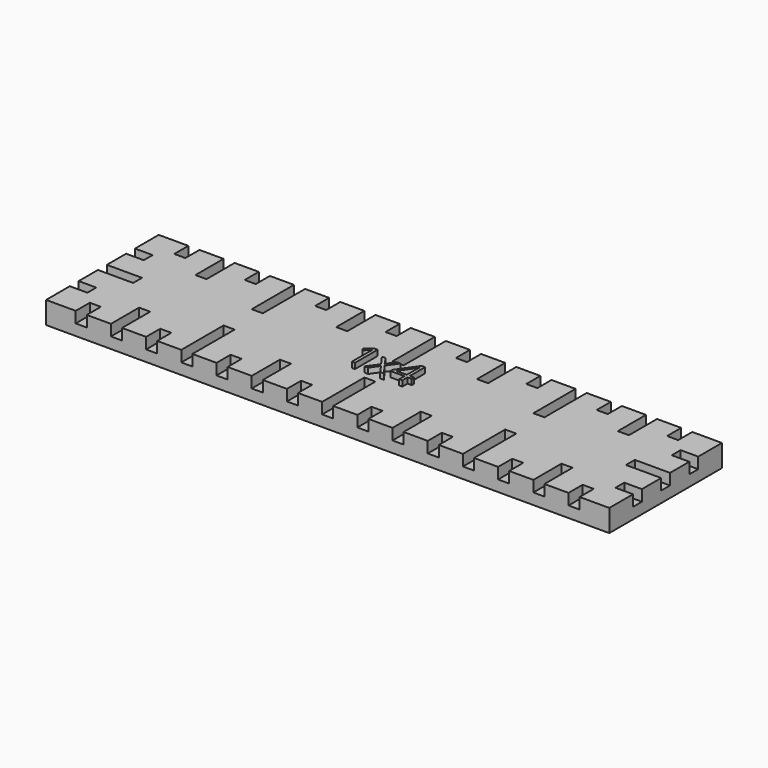
from build123d import *

# Parameters (mm, degrees)
F0_W         = 101.6
F0_H         = 25.4
F1_DEPTH     = 4
F2_W         = 2
F2_H         = 19.05
F2_H_2       = 6.35
F2_W_2       = 12.7
F2_H_3       = 2
F2_W_3       = 6.35
F2_H_4       = 12.7
F2_W_4       = 0.0030803442
F2_W_5       = 1.9969196558
F2_H_5       = 6.3500001535
F3_DEPTH     = 2
F4_TEXT_SIZE = 7.1658423015
F5_DEPTH     = 1


# Not quite as in the source:
# - ends of sketch curves that miss each other by under 0.0002 mm in the source are joined
# - Text() gives the source's letters only with a copy of the font that has no kerning and outlines rounded to 1/6400 em; it was checked with that copy


with BuildPart() as f1:
    # F0 (on Top) → F1 (new body)
    with BuildSketch(Plane.XY):
        Rectangle(F0_W, F0_H)
    extrude(amount=F1_DEPTH)

    # F2 (on face) → F3 (cut)
    with BuildSketch(Plane.XY.offset(4)):
        with Locations((0, -12.7)):
            Rectangle(F2_W, F2_H)
        with Locations((6.35, -12.7)):
            Rectangle(F2_W, F2_H_2)
        with Locations((-6.35, -12.7)):
            Rectangle(F2_W, F2_H_2)
        with Locations((-50.8, 0)):
            Rectangle(F2_W_2, F2_H_3)
        with Locations((-50.8, 6.35)):
            Rectangle(F2_W_3, F2_H_3)
        with Locations((-50.8, -6.35)):
            Rectangle(F2_W_3, F2_H_3)
        with Locations((0, 12.7)):
            Rectangle(F2_W, F2_H)
        with Locations((-6.35, 12.7)):
            Rectangle(F2_W, F2_H_2)
        with Locations((6.35, 12.7)):
            Rectangle(F2_W, F2_H_2)
        with Locations((50.8, 0)):
            Rectangle(F2_W_2, F2_H_3)
        with Locations((50.8, -6.35)):
            Rectangle(F2_W_3, F2_H_3)
        with Locations((50.8, 6.35)):
            Rectangle(F2_W_3, F2_H_3)
        with Locations((-12.7, 12.7000001177)):
            Rectangle(F2_W, F2_H_4)
        with Locations((-18.0515401721, 12.7000001177)):
            Rectangle(F2_W_4, F2_H_2)
        with Locations((-19.0515401721, 12.7000001177)):
            Rectangle(F2_W_5, F2_H_2)
        with Locations((-20.0515401721, 12.700000041)):
            Rectangle(F2_W_4, F2_H_5)
        with Locations((-12.7, -12.7000005066)):
            Rectangle(F2_W, F2_H_4)
        with Locations((-18.0515401721, -12.7000005066)):
            Rectangle(F2_W_4, F2_H_2)
        Polygon((-20.05, -15.8750005066), (-18.0530803442, -15.8750005066), (-18.0530803442, -9.5249999616), (-20.05, -9.5250005066), align=None)
        Polygon((-20.0530803442, -15.8749999616), (-20.05, -15.8749999616), (-20.05, -9.5250005066), (-20.0530803442, -9.5249999616), align=None)
        with Locations((12.700000225, -12.7)):
            Rectangle(F2_W, F2_H_4)
        with Locations((19.050000225, -12.7)):
            Rectangle(F2_W, F2_H_2)
        with Locations((12.700000225, 12.7)):
            Rectangle(F2_W, F2_H_4)
        with Locations((19.050000225, 12.7)):
            Rectangle(F2_W, F2_H_2)
        with Locations((25.3999939412, 12.6999999616)):
            Rectangle(F2_W, F2_H)
        with Locations((31.7499939412, 12.6999999616)):
            Rectangle(F2_W, F2_H_2)
        with Locations((38.0999941662, 12.6999999616)):
            Rectangle(F2_W, F2_H_4)
        with Locations((44.4499941662, 12.6999999616)):
            Rectangle(F2_W, F2_H_2)
        with Locations((25.3999939412, -12.6999999642)):
            Rectangle(F2_W, F2_H)
        with Locations((31.7499939412, -12.6999999642)):
            Rectangle(F2_W, F2_H_2)
        with Locations((38.0999941662, -12.6999999642)):
            Rectangle(F2_W, F2_H_4)
        with Locations((44.4499941662, -12.6999999642)):
            Rectangle(F2_W, F2_H_2)
        with Locations((-25.4030803442, -12.6999999616)):
            Rectangle(F2_W, F2_H)
        with Locations((-31.7530803442, -12.6999999616)):
            Rectangle(F2_W, F2_H_2)
        with Locations((-38.1030805692, -12.6999999616)):
            Rectangle(F2_W, F2_H_4)
        with Locations((-44.4530805692, -12.6999999616)):
            Rectangle(F2_W, F2_H_2)
        with Locations((-25.4030803442, 12.6999999642)):
            Rectangle(F2_W, F2_H)
        with Locations((-31.7530803442, 12.6999999642)):
            Rectangle(F2_W, F2_H_2)
        with Locations((-38.1030805692, 12.6999999642)):
            Rectangle(F2_W, F2_H_4)
        with Locations((-44.4530805692, 12.6999999642)):
            Rectangle(F2_W, F2_H_2)
    extrude(amount=-F3_DEPTH, mode=Mode.SUBTRACT)

    # F4 (on face) → F5 (join)
    with BuildSketch(Plane.XY.offset(4)):
        with Locations((-6.1346328078, -2.0106884258)):
            Text('1x4', F4_TEXT_SIZE, font='Open Sans', text_align=(TextAlign.LEFT, TextAlign.BOTTOM))
    extrude(amount=F5_DEPTH)


solid = f1.part
